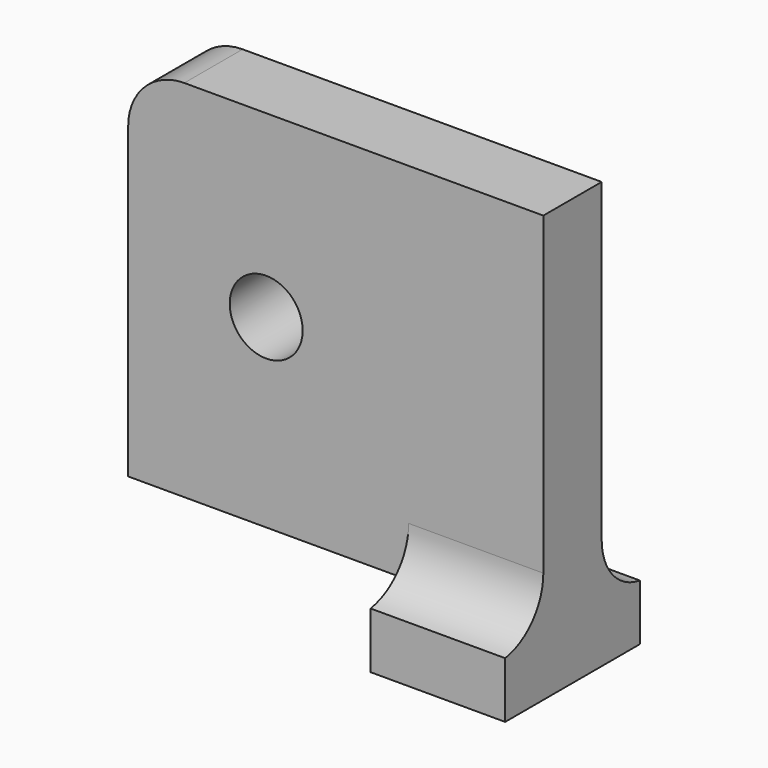
from build123d import *

# Parameters (mm, degrees)
F0_W        = 12
F0_H        = 15
F1_DEPTH    = 5
F2_W        = 12
F2_H        = 6.5
F3_DEPTH    = 33
F4_W        = 6.5
F4_H        = 33
F5_DEPTH    = 25
F6_T1_DEPTH = 12
F7_R        = 3.25
F8_DEPTH    = 25
F9_W        = 6.5
F9_H        = 0.5
F10_DEPTH   = 25
F11_R       = 5


# Not quite as in the source:
# - a fillet or chamfer that OpenCascade refuses, or shapes differently, is made with other operations: its cross-section is extruded or revolved along the edge and cut away or added


with BuildPart() as f1:
    # F0 (on Top) → F1 (new body)
    with BuildSketch(Plane.XY):
        Rectangle(F0_W, F0_H)
    extrude(amount=F1_DEPTH)

    # F2 (on face) → F3 (join)
    with BuildSketch(Plane.XY.offset(5)):
        Rectangle(F2_W, F2_H)
    extrude(amount=F3_DEPTH)

    # F4 (on face) → F5 (join)
    with BuildSketch(Plane(origin=(-6, 0, 0), x_dir=(0, -1, 0), z_dir=(-1, 0, 0))):
        with Locations((0, 21.5)):
            Rectangle(F4_W, F4_H)
    extrude(amount=F5_DEPTH)

    # F6: fillet of radius 5 on 2 edges, made by hand

    # F6_s2 → F6_t1 (join)
    with BuildSketch(Plane.YZ.offset(-6)):
        with BuildLine():
            ThreePointArc((-3.25, 9.9434299833), (-4.458562278, 6.6838287807), (-7.5, 5))
            Line((-7.5, 5), (-3.25, 5))
            Line((-3.25, 5), (-3.25, 9.9434299833))
        make_face()
        with BuildLine():
            ThreePointArc((7.5, 5), (4.458562278, 6.6838287807), (3.25, 9.9434299833))
            Line((3.25, 9.9434299833), (3.25, 5))
            Line((3.25, 5), (7.5, 5))
        make_face()
    extrude(amount=F6_T1_DEPTH)

    # F7 (on face) → F8 (cut)
    with BuildSketch(Plane.XZ.offset(3.25)):
        with Locations((-18.7, 22)):
            Circle(F7_R)
    extrude(amount=-F8_DEPTH, mode=Mode.SUBTRACT)

    # F9 (on face) → F10 (cut)
    with BuildSketch(Plane(origin=(-31, 0, 0), x_dir=(0, -1, 0), z_dir=(-1, 0, 0))):
        with Locations((0, 5.25)):
            Rectangle(F9_W, F9_H)
    extrude(amount=-F10_DEPTH, mode=Mode.SUBTRACT)

    # F11
    f11_edges = [f1.edges().sort_by_distance(p)[0] for p in [
        (-31, 0, 38),
    ]]
    fillet(f11_edges, radius=F11_R)


solid = f1.part
